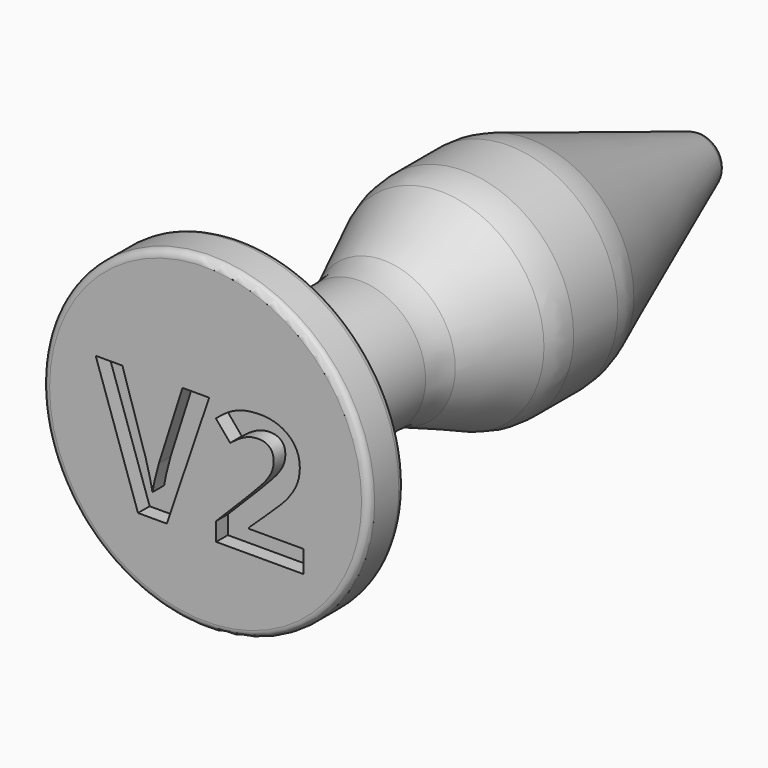
from build123d import *

# Parameters (mm, degrees)
F2_R         = 10
F3_R         = 3
F4_R         = 1
F5_R         = 2
F6_TEXT_SIZE = 23.9282153539
F7_DEPTH     = 2


# Not quite as in the source:
# - Text() gives the source's letters only with a copy of the font that has no kerning and outlines rounded to 1/6400 em; it was checked with that copy


with BuildPart() as f1:
    # F0 (on Top) → F1 (revolve)
    with BuildSketch(Plane.XY):
        Polygon((0, 74.8165398836), (0, 0), (22.3747331345, 0), (22.3747331345, 5.9277832573), (9, 8.9674954106), (9, 28.5380405618), (15, 42.1900498993), (15, 53.700563509), (2.9809876031, 85.1582282361), (0, 85.4954416847), align=None)
    revolve(axis=Axis((0, 38.0105182986, 0), (0, -1, 0)))

    # F2
    f2_edges = [f1.edges().sort_by_distance(p)[0] for p in [
        (-15, 42.19005, 0),
        (-9, 28.538041, 0),
        (-15, 53.700564, 0),
    ]]
    fillet(f2_edges, radius=F2_R)

    # F3
    f3_edges = [f1.edges().sort_by_distance(p)[0] for p in [
        (-9, 8.967495, 0),
    ]]
    fillet(f3_edges, radius=F3_R)

    # F4
    f4_edges = [f1.edges().sort_by_distance(p)[0] for p in [
        (-22.374733, 5.927783, 0),
        (-22.374733, 0, 0),
    ]]
    fillet(f4_edges, radius=F4_R)

    # F5
    f5_edges = [f1.edges().sort_by_distance(p)[0] for p in [
        (-2.980988, 85.158228, 0),
    ]]
    fillet(f5_edges, radius=F5_R)

    # F6 (on Front) → F7 (cut)
    with BuildSketch(Plane.XZ):
        with Locations((-15.0560001842, -11.2916806356)):
            Text('V2', F6_TEXT_SIZE, font='Open Sans', font_style=FontStyle.BOLD, text_align=(TextAlign.LEFT, TextAlign.BOTTOM))
    extrude(amount=-F7_DEPTH, mode=Mode.SUBTRACT)


solid = f1.part
